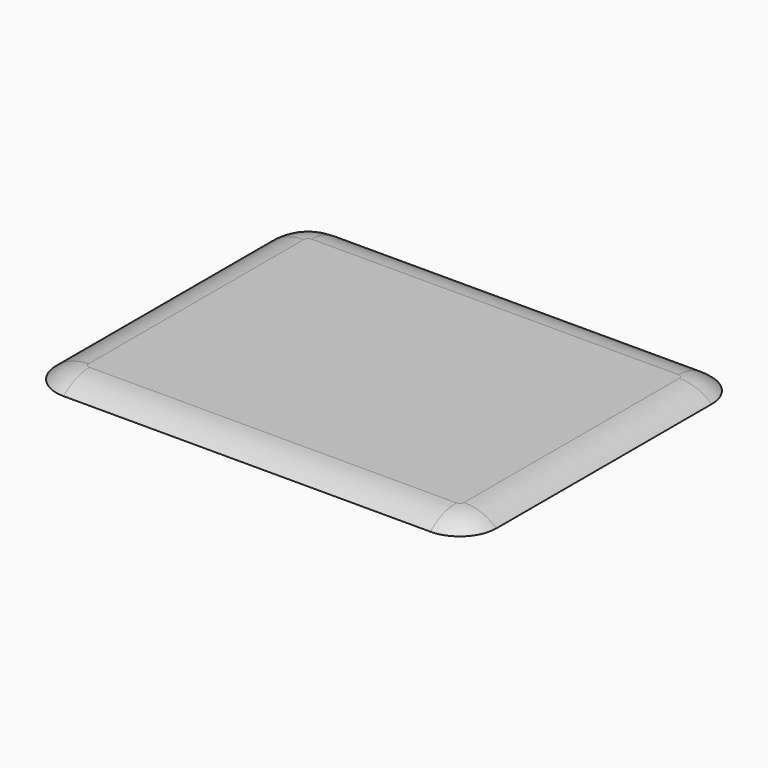
from build123d import *

# Parameters (mm, degrees)
F1_DEPTH     = 1.27
F2_T1_DEPTH  = 27.94
F2_T3_DEPTH  = 38.1
F2_T6_ANGLE  = 90
F2_T8_ANGLE  = 90
F2_T10_ANGLE = 90
F2_T12_ANGLE = 90


# Not quite as in the source:
# - a fillet or chamfer that OpenCascade refuses, or shapes differently, is made with other operations: its cross-section is extruded or revolved along the edge and cut away or added


with BuildPart() as f1:
    # F0 (on Top) → F1 (new body)
    with BuildSketch(Plane.XY):
        with BuildLine():
            ThreePointArc((22.86, 13.97), (21.7440768363, 16.6640768363), (19.05, 17.78))
            Line((19.05, 17.78), (-19.05, 17.78))
            ThreePointArc((-19.05, 17.78), (-21.7440768363, 16.6640768363), (-22.86, 13.97))
            Line((-22.86, 13.97), (-22.86, -13.97))
            ThreePointArc((-22.86, -13.97), (-21.7440768363, -16.6640768363), (-19.05, -17.78))
            Line((-19.05, -17.78), (19.05, -17.78))
            ThreePointArc((19.05, -17.78), (21.7440768363, -16.6640768363), (22.86, -13.97))
            Line((22.86, -13.97), (22.86, 13.97))
        make_face()
    extrude(amount=F1_DEPTH)

    # F2: fillet of radius 5.08 on 1 edges, made by hand

    # F2_s2 → F2_t1 (cut)
    with BuildSketch(Plane.XZ.offset(-13.97)):
        with BuildLine():
            ThreePointArc((-22.86, 0), (-21.2959470592, 0.9419048812), (-19.4998958349, 1.27))
            Line((-19.4998958349, 1.27), (-22.86, 1.27))
            Line((-22.86, 1.27), (-22.86, 0))
        make_face()
        with BuildLine():
            ThreePointArc((22.86, 0), (21.2959470592, 0.9419048812), (19.4998958349, 1.27))
            Line((19.4998958349, 1.27), (22.86, 1.27))
            Line((22.86, 1.27), (22.86, 0))
        make_face()
    extrude(amount=F2_T1_DEPTH, mode=Mode.SUBTRACT)

    # F2_s4 → F2_t3 (cut)
    with BuildSketch(Plane.YZ.offset(-19.05)):
        with BuildLine():
            ThreePointArc((-17.78, 0), (-16.2159470592, 0.9419048812), (-14.4198958349, 1.27))
            Line((-14.4198958349, 1.27), (-17.78, 1.27))
            Line((-17.78, 1.27), (-17.78, 0))
        make_face()
        with BuildLine():
            ThreePointArc((17.78, 0), (16.2159470592, 0.9419048812), (14.4198958349, 1.27))
            Line((14.4198958349, 1.27), (17.78, 1.27))
            Line((17.78, 1.27), (17.78, 0))
        make_face()
    extrude(amount=F2_T3_DEPTH, mode=Mode.SUBTRACT)

    # F2_s5 → F2_t6 (revolve, cut)
    with BuildSketch(Plane.YZ.offset(-19.05)):
        with BuildLine():
            ThreePointArc((17.78, 0), (16.2159470592, 0.9419048812), (14.4198958349, 1.27))
            Line((14.4198958349, 1.27), (17.78, 1.27))
            Line((17.78, 1.27), (17.78, 0))
        make_face()
    revolve(axis=Axis((-19.05, 13.97, 1.27), (0, 0, 1)), revolution_arc=F2_T6_ANGLE, mode=Mode.SUBTRACT)

    # F2_s7 → F2_t8 (revolve, cut)
    with BuildSketch(Plane.XZ.offset(13.97)):
        with BuildLine():
            ThreePointArc((-22.86, 0), (-21.2959470592, 0.9419048812), (-19.4998958349, 1.27))
            Line((-19.4998958349, 1.27), (-22.86, 1.27))
            Line((-22.86, 1.27), (-22.86, 0))
        make_face()
    revolve(axis=Axis((-19.05, -13.97, 1.27), (0, 0, 1)), revolution_arc=F2_T8_ANGLE, mode=Mode.SUBTRACT)

    # F2_s9 → F2_t10 (revolve, cut)
    with BuildSketch(Plane.YZ.offset(19.05)):
        with BuildLine():
            ThreePointArc((-17.78, 0), (-16.2159470592, 0.9419048812), (-14.4198958349, 1.27))
            Line((-14.4198958349, 1.27), (-17.78, 1.27))
            Line((-17.78, 1.27), (-17.78, 0))
        make_face()
    revolve(axis=Axis((19.05, -13.97, 1.27), (0, 0, 1)), revolution_arc=F2_T10_ANGLE, mode=Mode.SUBTRACT)

    # F2_s11 → F2_t12 (revolve, cut)
    with BuildSketch(Plane.XZ.offset(-13.97)):
        with BuildLine():
            ThreePointArc((22.86, 0), (21.2959470592, 0.9419048812), (19.4998958349, 1.27))
            Line((19.4998958349, 1.27), (22.86, 1.27))
            Line((22.86, 1.27), (22.86, 0))
        make_face()
    revolve(axis=Axis((19.05, 13.97, 1.27), (0, 0, 1)), revolution_arc=F2_T12_ANGLE, mode=Mode.SUBTRACT)


solid = f1.part
